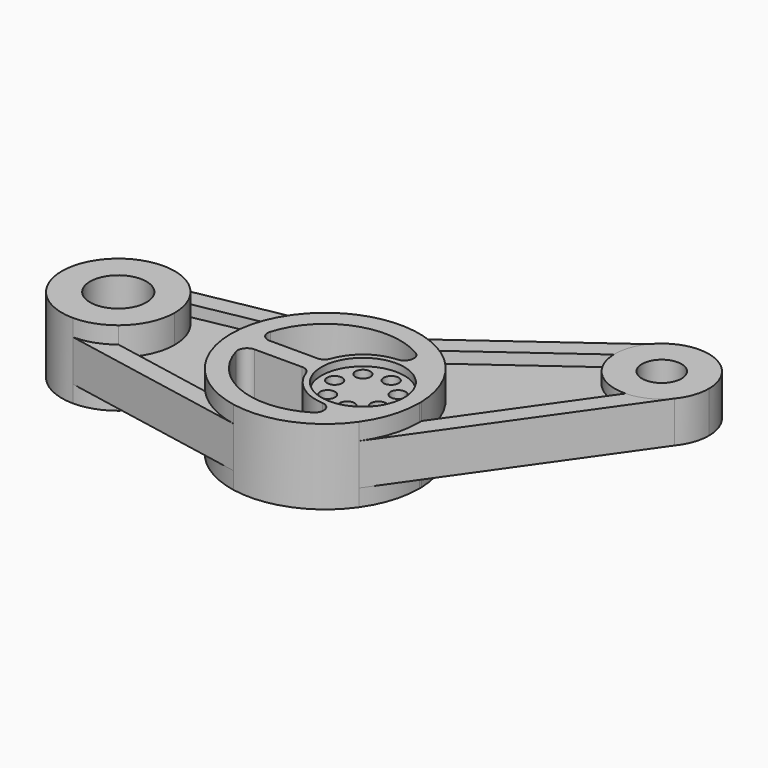
from build123d import *

# Parameters (mm, degrees)
F0_R     = 15
F1_DEPTH = 20
F0_R_2   = 22
F2_DEPTH = 11
F0_R_3   = 10.5
F3_DEPTH = 11
F0_R_4   = 4
F4_DEPTH = 16
F5_DEPTH = 5
F6_R     = 5


with BuildPart() as f1:
    # F0 (on Top) → F1 (new body, symmetric)
    with BuildSketch(Plane.XY):
        with BuildLine():
            ThreePointArc((-111.213639, -23.389584), (-102.948283, -12.969371), (-100, 0))
            ThreePointArc((-100, 0), (-102.948283, 12.969371), (-111.213639, 23.389584))
            ThreePointArc((-111.213639, 23.389584), (-120.042277, 28.299183), (-130, 30))
            ThreePointArc((-130, 30), (-160, 0), (-130, -30))
            ThreePointArc((-130, -30), (-120.042277, -28.299183), (-111.213639, -23.389584))
        make_face()
        with Locations((-130, 0)):
            Circle(F0_R, mode=Mode.SUBTRACT)
    extrude(amount=F1_DEPTH, both=True)


with BuildPart() as f1b:
    # F0 (on Top) → F1, piece 2 (new body, symmetric)
    with BuildSketch(Plane.XY):
        with BuildLine():
            ThreePointArc((-29.330441, 49.121715), (-44.385284, 43.650406), (-56.937382, 33.699107))
            ThreePointArc((-56.937382, 33.699107), (-70, 0), (-56.937382, -33.699107))
            ThreePointArc((-56.937382, -33.699107), (-44.385284, -43.650406), (-29.330441, -49.121715))
            ThreePointArc((-29.330441, -49.121715), (-1.201335, -46.331525), (20.919479, -28.73319))
            ThreePointArc((20.919479, -28.73319), (27.675853, -15.066951), (30, 0))
            ThreePointArc((30, 0), (29.993874, 0.782664), (29.975498, 1.565135))
            ThreePointArc((29.975498, 1.565135), (17.566054, 32.996842), (-12.002759, 49.356298))
            ThreePointArc((-12.002759, 49.356298), (-20.676841, 49.995419), (-29.330441, 49.121715))
        make_face()
        with BuildLine():
            Line((-59.68627, -5), (-24.494897, -5))
            ThreePointArc((-24.494897, -5), (-9.236251, -23.231265), (14.375, -20.453835))
            ThreePointArc((14.375, -20.453835), (-28.170536, -39.156639), (-59.68627, -5))
        make_face(mode=Mode.SUBTRACT)
        Circle(F0_R_2, mode=Mode.SUBTRACT)
        with BuildLine():
            ThreePointArc((14.375, 20.453835), (-9.236251, 23.231265), (-24.494897, 5))
            Line((-24.494897, 5), (-59.68627, 5))
            ThreePointArc((-59.68627, 5), (-28.170536, 39.156639), (14.375, 20.453835))
        make_face(mode=Mode.SUBTRACT)
    extrude(amount=F1_DEPTH, both=True)

    # F0 (on Top) → F4 (join, symmetric)
    with BuildSketch(Plane.XY):
        Circle(F0_R_2)
        with Locations((3.337814, -14.623919)):
            Circle(F0_R_4, mode=Mode.SUBTRACT)
        with Locations((-9.352347, -11.727472)):
            Circle(F0_R_4, mode=Mode.SUBTRACT)
        with Locations((-15, 0)):
            Circle(F0_R_4, mode=Mode.SUBTRACT)
        with Locations((-9.352347, 11.727472)):
            Circle(F0_R_4, mode=Mode.SUBTRACT)
        with Locations((3.337814, 14.623919)):
            Circle(F0_R_4, mode=Mode.SUBTRACT)
        with Locations((13.514533, -6.508256)):
            Circle(F0_R_4, mode=Mode.SUBTRACT)
        with Locations((13.514533, 6.508256)):
            Circle(F0_R_4, mode=Mode.SUBTRACT)
    extrude(amount=F4_DEPTH, both=True)

    # F6
    f6_edges = [f1b.edges().sort_by_distance(p)[0] for p in [
        (-59.68627, 5, -10),
        (-59.68627, 5, 10),
        (-24.494897, -5, -10),
        (-24.494897, -5, 10),
        (14.375, -20.453835, -10),
        (14.375, -20.453835, 10),
        (-59.68627, -5, -10),
        (-59.68627, -5, 10),
        (14.375, 20.453835, -10),
        (14.375, 20.453835, 10),
        (-24.494897, 5, -10),
        (-24.494897, 5, 10),
    ]]
    fillet(f6_edges, radius=F6_R)


with BuildPart() as f2:
    # F0 (on Top) → F2 (new body, symmetric)
    with BuildSketch(Plane.XY):
        with BuildLine():
            ThreePointArc((-130, 30), (-120.042277, 28.299183), (-111.213639, 23.389584))
            Line((-111.213639, 23.389584), (-56.937382, 33.699107))
            ThreePointArc((-56.937382, 33.699107), (-44.385284, 43.650406), (-29.330441, 49.121715))
            Line((-29.330441, 49.121715), (-130, 30))
        make_face()
    extrude(amount=F2_DEPTH, both=True)


with BuildPart() as f2b:
    # F0 (on Top) → F2, piece 2 (new body, symmetric)
    with BuildSketch(Plane.XY):
        with BuildLine():
            Line((-56.937382, -33.699107), (-111.213639, -23.389584))
            ThreePointArc((-111.213639, -23.389584), (-120.042277, -28.299183), (-130, -30))
            Line((-130, -30), (-29.330441, -49.121715))
            ThreePointArc((-29.330441, -49.121715), (-44.385284, -43.650406), (-56.937382, -33.699107))
        make_face()
    extrude(amount=F2_DEPTH, both=True)


with BuildPart() as f2c:
    # F0 (on Top) → F2, piece 3 (new body, symmetric)
    with BuildSketch(Plane.XY):
        with BuildLine():
            ThreePointArc((30, 0), (27.675853, -15.066951), (20.919479, -28.73319))
            Line((20.919479, -28.73319), (99.352339, 82.964527))
            ThreePointArc((99.352339, 82.964527), (91.005574, 76.2879), (80.633114, 73.707605))
            Line((80.633114, 73.707605), (29.975498, 1.565135))
            ThreePointArc((29.975498, 1.565135), (29.993874, 0.782664), (30, 0))
        make_face()
    extrude(amount=F2_DEPTH, both=True)


with BuildPart() as f2d:
    # F0 (on Top) → F2, piece 4 (new body, symmetric)
    with BuildSketch(Plane.XY):
        with BuildLine():
            Line((60.495041, 114.430547), (-29.330441, 49.121715))
            ThreePointArc((-29.330441, 49.121715), (-20.676841, 49.995419), (-12.002759, 49.356298))
            Line((-12.002759, 49.356298), (54.932799, 98.022701))
            ThreePointArc((54.932799, 98.022701), (56.247157, 106.723855), (60.495041, 114.430547))
        make_face()
    extrude(amount=F2_DEPTH, both=True)


with BuildPart() as f3:
    # F0 (on Top) → F3 (new body, symmetric)
    with BuildSketch(Plane.XY):
        with BuildLine():
            ThreePointArc((104.92369, 98.697537), (88.268861, 122.263574), (60.495041, 114.430547))
            ThreePointArc((60.495041, 114.430547), (56.247157, 106.723855), (54.932799, 98.022701))
            ThreePointArc((54.932799, 98.022701), (62.742206, 80.537233), (80.633114, 73.707605))
            ThreePointArc((80.633114, 73.707605), (91.005574, 76.2879), (99.352339, 82.964527))
            ThreePointArc((99.352339, 82.964527), (103.489727, 90.352366), (104.92369, 98.697537))
        make_face()
        with Locations((79.92369, 98.697537)):
            Circle(F0_R_3, mode=Mode.SUBTRACT)
    extrude(amount=F3_DEPTH, both=True)


with BuildPart() as f5:
    # F0 (on Top) → F5 (new body, symmetric)
    with BuildSketch(Plane.XY):
        with BuildLine():
            Line((54.932799, 98.022701), (-12.002759, 49.356298))
            ThreePointArc((-12.002759, 49.356298), (17.566054, 32.996842), (29.975498, 1.565135))
            Line((29.975498, 1.565135), (80.633114, 73.707605))
            ThreePointArc((80.633114, 73.707605), (62.742206, 80.537233), (54.932799, 98.022701))
        make_face()
    extrude(amount=F5_DEPTH, both=True)


with BuildPart() as f5b:
    # F0 (on Top) → F5, piece 2 (new body, symmetric)
    with BuildSketch(Plane.XY):
        with BuildLine():
            ThreePointArc((-111.213639, 23.389584), (-102.948283, 12.969371), (-100, 0))
            ThreePointArc((-100, 0), (-102.948283, -12.969371), (-111.213639, -23.389584))
            Line((-111.213639, -23.389584), (-56.937382, -33.699107))
            ThreePointArc((-56.937382, -33.699107), (-70, 0), (-56.937382, 33.699107))
            Line((-56.937382, 33.699107), (-111.213639, 23.389584))
        make_face()
    extrude(amount=F5_DEPTH, both=True)


solid = Compound([f1.part, f1b.part, f2.part, f2b.part, f2c.part, f2d.part, f3.part, f5.part, f5b.part])
